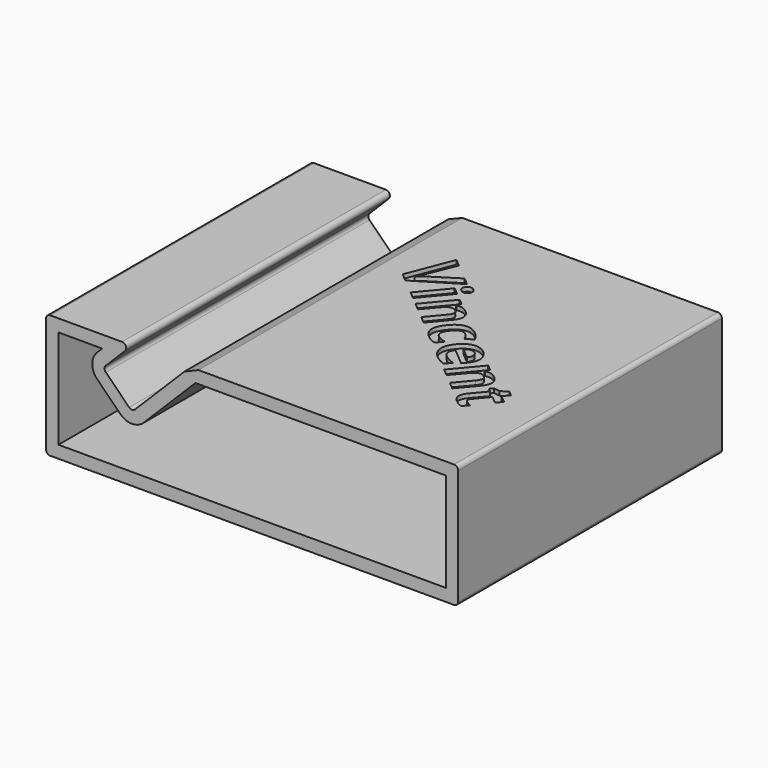
from build123d import *

# Parameters (mm, degrees)
F0_W         = 100
F0_H         = 80
F1_DEPTH     = 30
F3_DEPTH     = 80
F4_R         = 1
F5_T         = -3
F6_TEXT_SIZE = 15.6205507871
F7_DEPTH     = 1
F8_SIZE      = 2


# Not quite as in the source:
# - Text() gives the source's letters only with a copy of the font that has no kerning and outlines rounded to 1/6400 em; it was checked with that copy


with BuildPart() as f1:
    # F0 (on Top) → F1 (new body)
    with BuildSketch(Plane.XY):
        with Locations((4.8498727381, 0.9492458403)):
            Rectangle(F0_W, F0_H)
    extrude(amount=F1_DEPTH)

    # F2 (on face) → F3 (cut)
    with BuildSketch(Plane.XZ.offset(39.0507541597)):
        Polygon((-24.2922628856, 15.8578643763), (-10.1501272619, 30), (-24.2922628856, 30), (-31.3633306975, 22.9289321881), align=None)
    extrude(amount=-F3_DEPTH, mode=Mode.SUBTRACT)

    # F4
    f4_edges = [f1.edges().sort_by_distance(p)[0] for p in [
        (-24.292263, 0.949246, 15.857864),
        (-31.363331, 0.949246, 22.928932),
        (-24.292263, 0.949246, 30),
        (-45.150127, 0.949246, 30),
        (-45.150127, 0.949246, 0),
        (54.849873, 0.949246, 0),
        (54.849873, 0.949246, 30),
    ]]
    fillet(f4_edges, radius=F4_R)

    # F5
    f5_openings = [f1.faces().sort_by_distance(p)[0] for p in [
        (6.268652, -39.050754, 14.494062),
        (6.268652, 40.949246, 14.494062),
    ]]
    offset(amount=F5_T, openings=f5_openings)

    # F6 (on face) → F7 (cut)
    with BuildSketch(Plane.XY.offset(30)):
        with Locations(Location((-5.4043644659, 18.2516435255), (0, 0, -40))):
            Text('Vincent', F6_TEXT_SIZE, font='Open Sans', font_style=FontStyle.BOLD, text_align=(TextAlign.LEFT, TextAlign.BOTTOM))
    extrude(amount=-F7_DEPTH, mode=Mode.SUBTRACT)

    # F8
    f8_edges = [f1.edges().sort_by_distance(p)[0] for p in [
        (-10.150127, 0.949246, 30),
    ]]
    chamfer(f8_edges, length=F8_SIZE)


solid = f1.part
